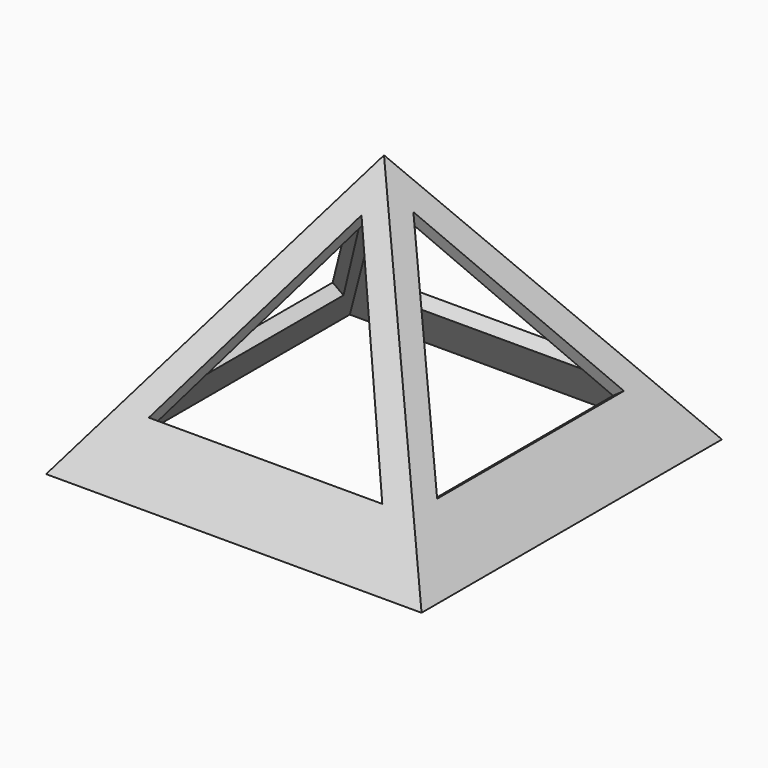
from build123d import *

# Parameters (mm, degrees)
F2_W      = 90
F2_H      = 90
F6_W      = 82
F6_H      = 82
F12_DEPTH = 5
F13_DEPTH = 10.1
F14_DEPTH = 10
F15_DEPTH = 10
F16_W     = 1.180001
F16_H     = 1.870001
F16_W_2   = 1.18
F16_H_2   = 4.060001
F16_W_3   = 10.110001
F16_H_3   = 1.18
F16_W_4   = 6.670001
F17_DEPTH = 2


# Not quite as in the source:
# - the dataset's text gives a spline's control points without its knots; the knots are read off the source's solid


with BuildPart() as f3:
    # F2 (on Top) → F3 section 0
    with BuildSketch(Plane.XY, mode=Mode.PRIVATE) as f3_s0:
        Rectangle(F2_W, F2_H)
    loft([f3_s0.sketch, Vertex(0, 0, 63.6368)])

    # F6 (on face) → F7 section 0
    with BuildSketch(Plane.XY, mode=Mode.PRIVATE) as f7_s0:
        Rectangle(F6_W, F6_H)
    loft([f7_s0.sketch, Vertex(0, 0, 58.6368)], mode=Mode.SUBTRACT)

    # F8 (on face) → F12 (cut, symmetric)
    with BuildSketch(Plane(origin=(29.9991167733, 0, 21.2135156827), x_dir=(0, 1, 0), z_dir=(0.8164845616, 0, 0.5773672666))):
        Polygon((0.1463476627, 39.9593571873), (-28.0024763197, -8.9000007138), (27.9615262598, -8.9000007138), align=None)
    extrude(amount=F12_DEPTH, both=True, mode=Mode.SUBTRACT)

    # F9 (on face) → F13 (cut)
    with BuildSketch(Plane(origin=(0, 29.9991167733, 21.2135156827), x_dir=(-1, 0, 0), z_dir=(0, 0.8164845616, 0.5773672666))):
        Polygon((0.1463476627, 39.9593571873), (-27.835653627, -8.5054690465), (28.1283489525, -8.5054690465), align=None)
    extrude(amount=-F13_DEPTH, mode=Mode.SUBTRACT)

    # F10 (on face) → F14 (cut)
    with BuildSketch(Plane(origin=(-29.9991167733, 0, 21.2135156827), x_dir=(0, -1, 0), z_dir=(-0.8164845616, 0, 0.5773672666))):
        Polygon((0.1463476627, 39.9593571873), (-28.9770383388, -9.5114903525), (26.9869642407, -9.5114903525), align=None)
    extrude(amount=-F14_DEPTH, mode=Mode.SUBTRACT)

    # F11 (on face) → F15 (cut)
    with BuildSketch(Plane(origin=(0, -29.9991167733, 21.2135156827), x_dir=(1, 0, 0), z_dir=(0, -0.8164845616, 0.5773672666))):
        Polygon((0.1463476627, 39.9593571873), (-28.0361250043, -9.3999961391), (27.9278775752, -9.3999961391), align=None)
    extrude(amount=-F15_DEPTH, mode=Mode.SUBTRACT)

    # F16 (on face) → F17 (cut)
    with BuildSketch(Plane(origin=(-29.9991167733, 0, 21.2135156827), x_dir=(0, -1, 0), z_dir=(-0.8164845616, 0, 0.5773672666))):
        Polygon((21.9697801374, -21.1938021154), (23.5597841374, -21.1938021154), (28.7397811374, -15.0950853876), (28.7397811374, -19.0038021154), (29.9197811374, -19.0038021154), (29.9197811374, -14.9538011154), (28.8597821374, -14.9538011154), (28.7397811374, -14.9538011154), (22.2197811374, -14.9538011154), (21.2197821374, -16.1338011154), (26.2597841374, -16.1338011154), align=None)
        with Locations((31.4797826374, -18.0688016154)):
            Rectangle(F16_W, F16_H)
        with Locations((33.6297791374, -19.1638016154)):
            Rectangle(F16_W_2, F16_H_2)
        Polygon((12.0897811374, -21.1938021154), (20.2597801374, -21.1938021154), (20.8297821374, -20.0438011154), (18.3297821374, -14.9538011154), (13.9597791374, -14.9538011154), (11.4997811374, -19.9838021154), align=None)
        Polygon((19.3697831374, -20.0138021154), (12.9197831374, -20.0138021154), (14.8197791374, -16.1338011154), (17.4797821374, -16.1338011154), align=None, mode=Mode.SUBTRACT)
        with BuildLine():
            Line((5.2997801374, -14.9538011154), (5.2997801374, -16.6038011154))
            add(Edge.make_bspline(
                [(4.1407171374, -16.7288011154), (4.3252931374, -16.7141861154), (4.7128221374, -16.6835011154), (5.0980381374, -16.6311951154), (5.2997801374, -16.6038011154)],
                knots=[0, 0, 0, 0, 0.555346, 1.165986, 1.165986, 1.165986, 1.165986], degree=3))
            add(Edge.make_bspline(
                [(3.2325931374, -16.7738011154), (3.3718421374, -16.7690131154), (3.6747741374, -16.7585981154), (3.9772701374, -16.7392531154), (4.1407171374, -16.7288011154)],
                knots=[0, 0, 0, 0, 0.417971, 0.909282, 0.909282, 0.909282, 0.909282], degree=3))
            add(Edge.make_bspline(
                [(2.4297801374, -16.7638011154), (2.5552081374, -16.7691171154), (2.8227031374, -16.7804551154), (3.0904121374, -16.7761091154), (3.2325931374, -16.7738011154)],
                knots=[0, 0, 0, 0, 0.376537, 0.803027, 0.803027, 0.803027, 0.803027], degree=3))
            Line((2.4297801374, -16.7638011154), (1.2497801374, -16.7638011154))
            Line((1.2497801374, -16.7638011154), (1.2497801374, -21.1938021154))
            Line((1.2497801374, -21.1938021154), (10.6597801374, -21.1938021154))
            Line((10.6597801374, -21.1938021154), (10.6597801374, -20.0138021154))
            Line((10.6597801374, -20.0138021154), (6.4797801374, -20.0138021154))
            Line((6.4797801374, -20.0138021154), (6.4797801374, -17.6491141154))
            add(Edge.make_bspline(
                [(8.6047791374, -17.0530201154), (8.2523501374, -17.1763541154), (7.5565571374, -17.4198491154), (6.8355751374, -17.5733591154), (6.4797801374, -17.6491141154)],
                knots=[0, 0, 0, 0, 1.118887, 2.208999, 2.208999, 2.208999, 2.208999], degree=3))
            add(Edge.make_bspline(
                [(10.6597801374, -16.1361451154), (10.3259741374, -16.3048751154), (9.6557671374, -16.6436461154), (8.9560111374, -16.9162101154), (8.6047791374, -17.0530201154)],
                knots=[0, 0, 0, 0, 1.121359, 2.251432, 2.251432, 2.251432, 2.251432], degree=3))
            Line((10.6597801374, -16.1361451154), (10.6597801374, -14.9538011154))
            add(Edge.make_bspline(
                [(8.5247801374, -15.8638011154), (8.8834781374, -15.7390181154), (9.6157961374, -15.4842611154), (10.3070901374, -15.1330071154), (10.6597801374, -14.9538011154)],
                knots=[0, 0, 0, 0, 1.137935, 2.323212, 2.323212, 2.323212, 2.323212], degree=3))
            add(Edge.make_bspline(
                [(6.4797801374, -16.4038011154), (6.8146711374, -16.3298001154), (7.5036441374, -16.1775551154), (8.1781381374, -15.9703101154), (8.5247801374, -15.8638011154)],
                knots=[0, 0, 0, 0, 1.028459, 2.115858, 2.115858, 2.115858, 2.115858], degree=3))
            Line((6.4797801374, -16.4038011154), (6.4797801374, -14.9538011154))
            Line((6.4797801374, -14.9538011154), (5.2997801374, -14.9538011154))
        make_face()
        with BuildLine():
            Line((5.2997801374, -20.0138021154), (2.4297801374, -20.0138021154))
            Line((2.4297801374, -20.0138021154), (2.4297801374, -17.9538021154))
            add(Edge.make_bspline(
                [(3.2525921374, -17.9638011154), (3.1087451374, -17.9660571154), (2.8343741374, -17.9703591154), (2.5602071374, -17.9591391154), (2.4297801374, -17.9538021154)],
                knots=[0, 0, 0, 0, 0.431492, 0.823018, 0.823018, 0.823018, 0.823018], degree=3))
            add(Edge.make_bspline(
                [(4.1557951374, -17.9288011154), (3.9935791374, -17.9363501154), (3.6926011374, -17.9503551154), (3.3914391374, -17.9595581154), (3.2525921374, -17.9638011154)],
                knots=[0, 0, 0, 0, 0.487164, 0.903894, 0.903894, 0.903894, 0.903894], degree=3))
            add(Edge.make_bspline(
                [(5.2997801374, -17.8238011154), (5.1009381374, -17.8479581154), (4.7206281374, -17.8941601154), (4.3382501374, -17.9176111154), (4.1557951374, -17.9288011154)],
                knots=[0, 0, 0, 0, 0.600755, 1.14902, 1.14902, 1.14902, 1.14902], degree=3))
            Line((5.2997801374, -17.8238011154), (5.2997801374, -20.0138021154))
        make_face(mode=Mode.SUBTRACT)
        Polygon((-7.2802218626, -14.9538011154), (-9.6202208626, -19.7238021154), (-11.9602208626, -14.9538011154), (-13.3902208626, -14.9538011154), (-10.3302198626, -21.1938021154), (-8.9002208626, -21.1938021154), (-6.4202218626, -16.1338011154), (-5.8402208626, -16.1338011154), (-5.8402208626, -21.1938021154), (-4.6602208626, -21.1938021154), (-4.6602208626, -16.1338011154), (-3.9402198626, -16.1338011154), (-3.9402198626, -14.9538011154), align=None)
        with Locations((-18.7952213626, -15.5438011154)):
            Rectangle(F16_W_3, F16_H_3)
        with Locations((-18.7952213626, -18.0738011154)):
            Rectangle(F16_W_4, F16_H_3)
        with Locations((-18.7952213626, -20.6038021154)):
            Rectangle(F16_W_3, F16_H_3)
        Polygon((-33.1302218626, -18.0738021154), (-30.4802218626, -21.1938021154), (-27.3102218626, -21.1938021154), (-24.6602208626, -18.0738021154), (-26.2502218626, -18.0738021154), (-28.3002218626, -20.4938021154), (-28.3002218626, -14.9538011154), (-29.4802218626, -14.9538011154), (-29.4802218626, -20.4938021154), (-31.5402218626, -18.0738021154), align=None)
    extrude(amount=-F17_DEPTH, mode=Mode.SUBTRACT)


solid = f3.part
